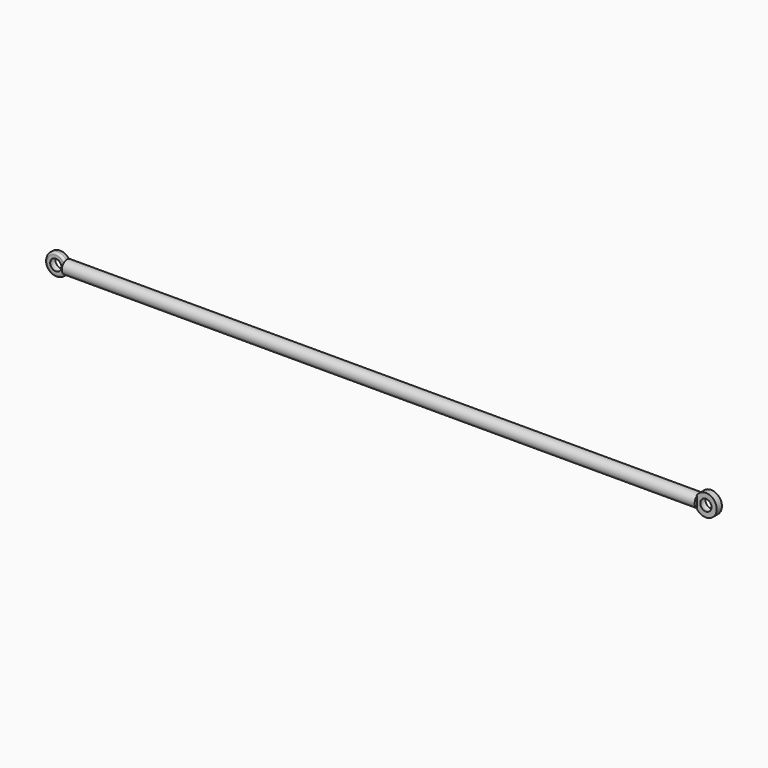
from build123d import *

# Parameters (mm, degrees)
F1_R         = 5
F1_R_2       = 2
F2_DEPTH     = 1.5
F5_R         = 3
F6_DEPTH     = 146
F9_T4_ANGLE  = 354.9348896549
F9_T9_ANGLE  = 354.9348896549
F9_S10_R     = 3
F9_T11_DEPTH = 9
F9_T15_ANGLE = 354.9348896549
F9_T20_ANGLE = 354.9348896549
F9_S21_R     = 3
F9_T22_DEPTH = 9


# Not quite as in the source:
# - a fillet or chamfer that OpenCascade refuses, or shapes differently, is made with other operations: its cross-section is extruded or revolved along the edge and cut away or added


with BuildPart() as f2:
    # F1 (on Front) → F2 (new body, symmetric)
    with BuildSketch(Plane.XZ):
        Circle(F1_R)
        Circle(F1_R_2, mode=Mode.SUBTRACT)
    extrude(amount=F2_DEPTH, both=True)

    # F0 (on Top) → F3 (revolve, cut)
    with BuildSketch(Plane.XY):
        with BuildLine():
            Line((1.5, 2.5980762114), (1.5, -2.5980762114))
            ThreePointArc((1.5, -2.5980762114), (3, 0), (1.5, 2.5980762114))
        make_face()
    revolve(axis=Axis((0, 0.5133161101, 0), (0, -1, 0)), mode=Mode.SUBTRACT)

    # F5 (on offset) → F6 (join)
    with BuildSketch(Plane.YZ.offset(4)):
        Circle(F5_R)
    extrude(amount=F6_DEPTH)

    # F8: F2 across plane


with BuildPart() as f2_1:
    add(f2.part)
    add(f2.part.mirror(Plane.YZ.offset(150)))

    # F9: fillet of radius 1 on 2 edges, made by hand


with BuildPart() as f9_tool2:
    # F9_s3 → F9_t4 (revolve)
    with BuildSketch(Plane(origin=(0, 0, 0), x_dir=(0, 1, 0), z_dir=(0.0441870344, 0, -0.999023276))):
        with BuildLine():
            ThreePointArc((-0.5, 5), (-1.2071067812, 4.7071067812), (-1.5, 4))
            Line((-1.5, 4), (-1.5, 5))
            Line((-1.5, 5), (-0.5, 5))
        make_face()
    revolve(axis=Axis((0, -1.5, 0), (0, -1, 0)), revolution_arc=F9_T4_ANGLE)

    split(bisect_by=Plane.YZ.offset(4), keep=Keep.BOTTOM)


with BuildPart() as f2_2:
    add(f2_1.part)

    # F9_t1: cut F9_tool2
    add(f9_tool2.part, mode=Mode.SUBTRACT)


with BuildPart() as f9_tool7:
    # F9_s8 → F9_t9 (revolve)
    with BuildSketch(Plane(origin=(0, 0, 0), x_dir=(0, 1, 0), z_dir=(0.0441870344, 0, -0.999023276))):
        with BuildLine():
            ThreePointArc((-0.5, 5), (-1.2071067812, 4.7071067812), (-1.5, 4))
            Line((-1.5, 4), (-1.5, 5))
            Line((-1.5, 5), (-0.5, 5))
        make_face()
    revolve(axis=Axis((0, -1.5, 0), (0, -1, 0)), revolution_arc=F9_T9_ANGLE)

    # F9_s10 → F9_t11 (cut, symmetric)
    with BuildSketch(Plane.YZ):
        Circle(F9_S10_R)
    extrude(amount=F9_T11_DEPTH, both=True, mode=Mode.SUBTRACT)


with BuildPart() as f2_3:
    add(f2_2.part)

    # F9_t6: cut F9_tool7
    add(f9_tool7.part, mode=Mode.SUBTRACT)


with BuildPart() as f9_tool13:
    # F9_s14 → F9_t15 (revolve)
    with BuildSketch(Plane(origin=(0, 0, 0), x_dir=(0, 1, 0), z_dir=(0.0441870344, 0, -0.999023276))):
        with BuildLine():
            ThreePointArc((0.5, 5), (1.2071067812, 4.7071067812), (1.5, 4))
            Line((1.5, 4), (1.5, 5))
            Line((1.5, 5), (0.5, 5))
        make_face()
    revolve(axis=Axis((0, 1.5, 0), (0, -1, 0)), revolution_arc=F9_T15_ANGLE)

    split(bisect_by=Plane.YZ.offset(4), keep=Keep.BOTTOM)


with BuildPart() as f2_4:
    add(f2_3.part)

    # F9_t12: cut F9_tool13
    add(f9_tool13.part, mode=Mode.SUBTRACT)


with BuildPart() as f9_tool18:
    # F9_s19 → F9_t20 (revolve)
    with BuildSketch(Plane(origin=(0, 0, 0), x_dir=(0, 1, 0), z_dir=(0.0441870344, 0, -0.999023276))):
        with BuildLine():
            ThreePointArc((0.5, 5), (1.2071067812, 4.7071067812), (1.5, 4))
            Line((1.5, 4), (1.5, 5))
            Line((1.5, 5), (0.5, 5))
        make_face()
    revolve(axis=Axis((0, 1.5, 0), (0, -1, 0)), revolution_arc=F9_T20_ANGLE)

    # F9_s21 → F9_t22 (cut, symmetric)
    with BuildSketch(Plane.YZ):
        Circle(F9_S21_R)
    extrude(amount=F9_T22_DEPTH, both=True, mode=Mode.SUBTRACT)


with BuildPart() as f2_5:
    add(f2_4.part)

    # F9_t17: cut F9_tool18
    add(f9_tool18.part, mode=Mode.SUBTRACT)


solid = f2_5.part
